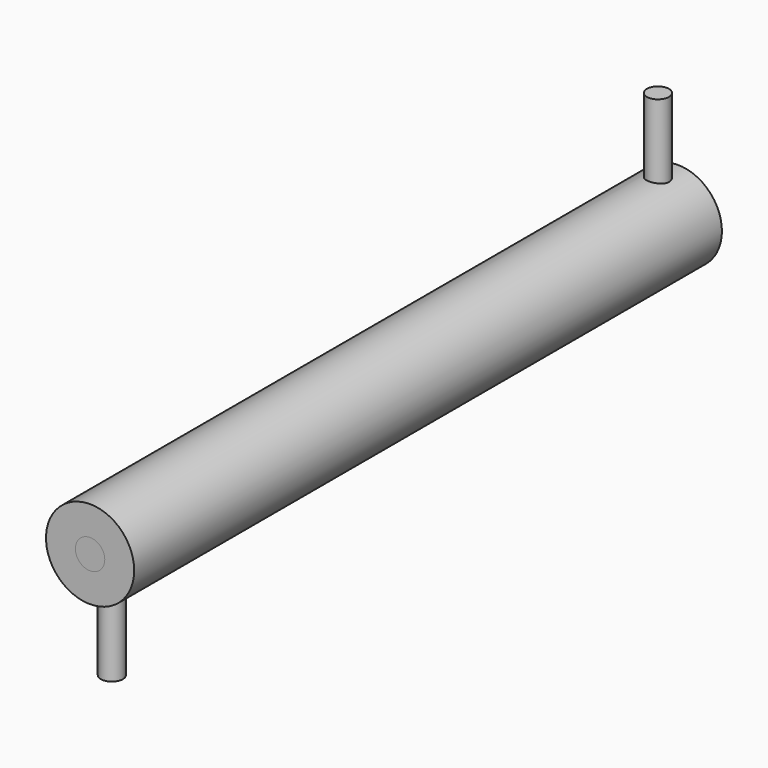
from build123d import *

# Parameters (mm, degrees)
F0_R     = 60
F2_DEPTH = 1000
F1_R     = 20
F3_R     = 15
F4_DEPTH = 160
F5_R     = 15
F6_DEPTH = 160


with BuildPart() as f2:
    # F0 (on Front) → F2 (new body)
    with BuildSketch(Plane.XZ):
        Circle(F0_R)
    extrude(amount=F2_DEPTH)

    # F3 (on Top) → F4 (join)
    with BuildSketch(Plane.XY):
        with Locations((0, -33.885266772)):
            Circle(F3_R)
    extrude(amount=F4_DEPTH)

    # F5 (on Top) → F6 (join)
    with BuildSketch(Plane.XY):
        with Locations((0, -962.9562497139)):
            Circle(F5_R)
    extrude(amount=-F6_DEPTH)


with BuildPart() as f2b:
    # F1 (on Front) → F2, piece 2 (new body)
    with BuildSketch(Plane.XZ):
        Circle(F1_R)
    extrude(amount=F2_DEPTH)


solid = Compound([f2.part, f2b.part])
